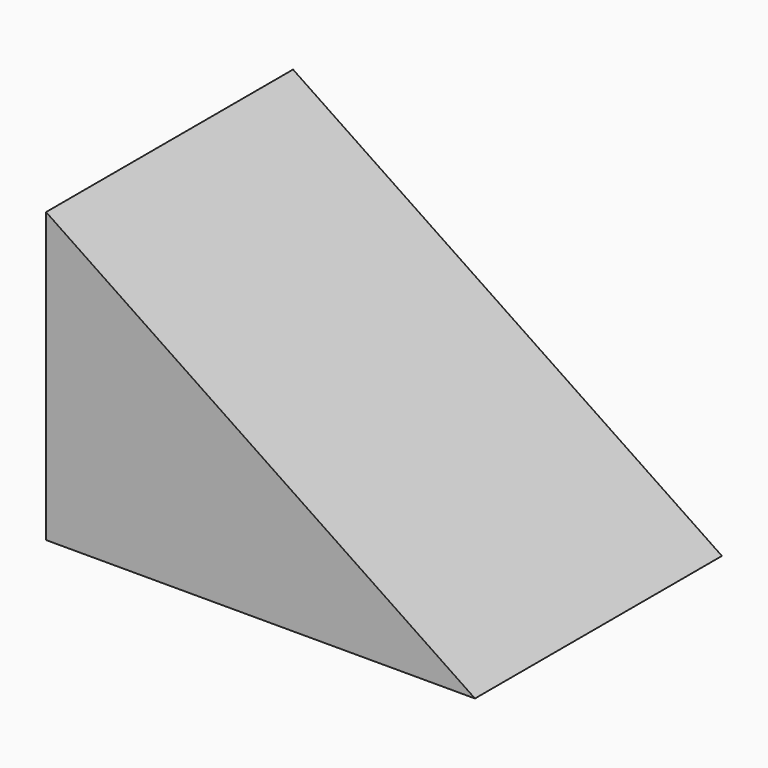
from build123d import *

# Parameters (mm, degrees)
F1_DEPTH = 41.387995705


with BuildPart() as f1:
    # F0 (on Front) → F1 (new body)
    with BuildSketch(Plane.XZ):
        Polygon((0, 0), (-57.4960261583, 38.7146770954), (-57.4960261583, 0), align=None)
    extrude(amount=-F1_DEPTH)


solid = f1.part
